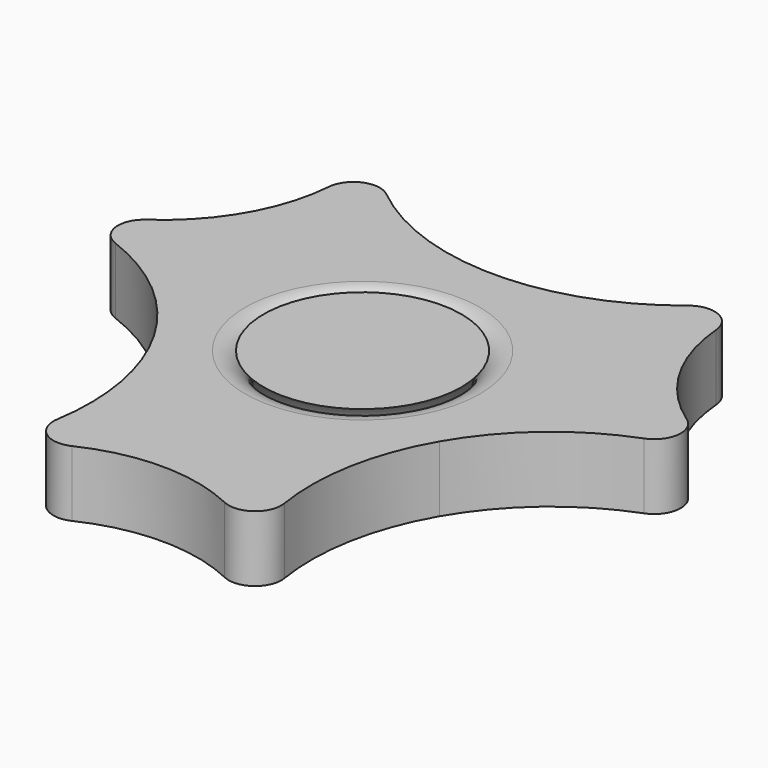
from build123d import *

# Parameters (mm, degrees)
F0_R     = 7.5
F0_R_2   = 6.7
F1_DEPTH = 5
F2_R     = 2
F3_R     = 2.2


# Not quite as in the source:
# - a feature names something its author has since deleted; it is built from what else it names


with BuildPart() as f1:
    # F0 (on Top) → F1 (new body)
    with BuildSketch(Plane.XY):
        with BuildLine():
            ThreePointArc((12.5, 0), (8.8388347698, 8.8388347598), (1.42e-08, 12.5))
            ThreePointArc((1.42e-08, 12.5), (-10.8253174308, 6.2500002019), (-10.8253177733, -6.2499996085))
            ThreePointArc((-10.8253177733, -6.2499996085), (-4.25e-08, -12.5), (10.8253177308, -6.2499996822))
            ThreePointArc((10.8253177308, -6.2499996822), (12.0740728761, -3.2352378865), (12.5, 0))
        make_face()
        Circle(F0_R, mode=Mode.SUBTRACT)
        Circle(F0_R)
        Circle(F0_R_2, mode=Mode.SUBTRACT)
        with BuildLine():
            ThreePointArc((26.773933784, 2.8198878343), (16.4544826719, 9.5), (15.8290613924, 21.776962899))
            ThreePointArc((15.8290613924, 21.776962899), (9.1736201366, 14.9901270648), (1.42e-08, 12.5))
            ThreePointArc((1.42e-08, 12.5), (8.8388347698, 8.8388347598), (12.5, 0))
            ThreePointArc((12.5, 0), (12.0740728761, -3.2352378865), (10.8253177308, -6.2499996822))
            ThreePointArc((10.8253177308, -6.2499996822), (17.5686410658, 0.4495246378), (26.773933784, 2.8198878343))
        make_face()
        with BuildLine():
            ThreePointArc((-10.8253177733, -6.2499996085), (-10.8253174308, 6.2500002019), (1.42e-08, 12.5))
            ThreePointArc((1.42e-08, 12.5), (-9.1736201244, 14.9901270577), (-15.8290613924, 21.7769628991))
            ThreePointArc((-15.8290613924, 21.7769628991), (-14.9449484341, 19.0761000413), (-14.645825623, 16.25))
            ThreePointArc((-14.645825623, 16.25), (-18.1265806458, 7.2020869762), (-26.773933784, 2.8198878343))
            ThreePointArc((-26.773933784, 2.8198878343), (-17.5686411027, 0.4495246588), (-10.8253177733, -6.2499996085))
        make_face()
        with BuildLine():
            ThreePointArc((10.9448723917, -24.5968507334), (8.3950207746, -15.4396514248), (10.8253177308, -6.2499996822))
            ThreePointArc((10.8253177308, -6.2499996822), (-4.25e-08, -12.5), (-10.8253177733, -6.2499996085))
            ThreePointArc((-10.8253177733, -6.2499996085), (-8.3950207743, -15.4396513823), (-10.9448723917, -24.5968507334))
            ThreePointArc((-10.9448723917, -24.5968507334), (0, -19), (10.9448723917, -24.5968507334))
        make_face()
    extrude(amount=F1_DEPTH)

    # F2
    f2_edges = [f1.edges().sort_by_distance(p)[0] for p in [
        (10.944872, -24.596851, 2.5),
        (-10.944872, -24.596851, 2.5),
        (26.773934, 2.819888, 2.5),
        (15.829061, 21.776963, 2.5),
        (-26.773934, 2.819888, 2.5),
        (-15.829061, 21.776963, 2.5),
    ]]
    fillet(f2_edges, radius=F2_R)

    # F3
    f3_edges = [f1.edges().sort_by_distance(p)[0] for p in [
        (-6.7, 0, 5),
        (-6.7, 0, 0),
    ]]
    fillet(f3_edges, radius=F3_R)


with BuildPart() as f5:
    # F4 (on Front) → F5 (revolve)
    with BuildSketch(Plane.XZ):
        with BuildLine():
            Line((7.5, 5), (0, 5))
            Line((0, 5), (0, 0))
            Line((0, 0), (7.5, 0))
            ThreePointArc((7.5, 0), (6.5, 2.5), (7.5, 5))
        make_face()
    revolve(axis=Axis((0, 0, 5.3585310292), (0, 0, 1)))


solid = Compound([f1.part, f5.part])
